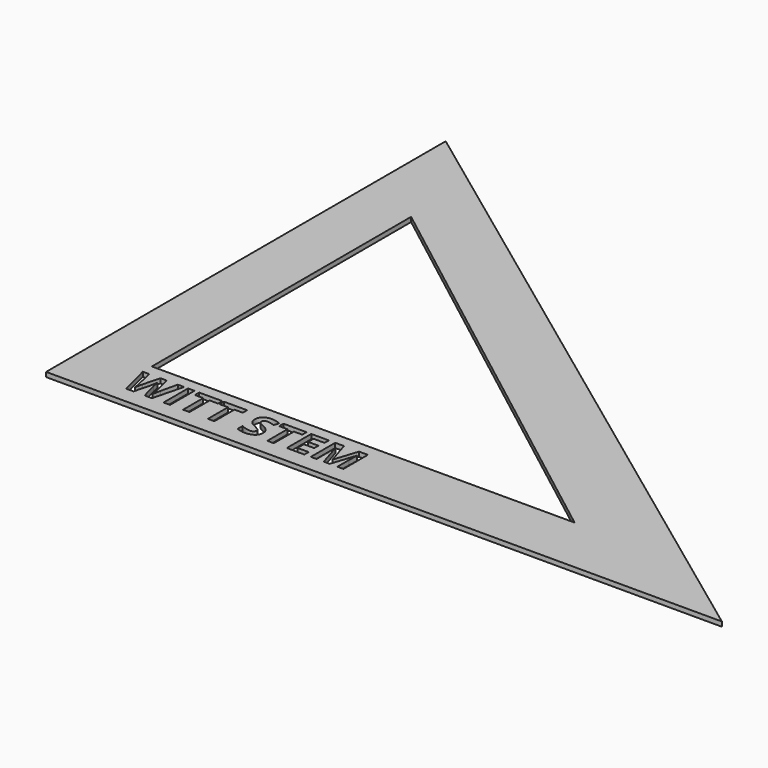
from build123d import *

# Parameters (mm, degrees)
F1_DEPTH     = 2
F2_SCALE     = 0.75
F3_TEXT_SIZE = 13.8751121122
F4_DEPTH     = 1.501


# Not quite as in the source:
# - Text() gives the source's letters only with a copy of the font that has no kerning and outlines rounded to 1/6400 em; it was checked with that copy


with BuildPart() as f1:
    # F0 (on Top) → F1 (new body)
    with BuildSketch(Plane.XY):
        Polygon((-110.3935540405, 109.5033976257), (-110.3935540405, -106.3966023743), (181.7064459595, -106.3966023743), align=None)
        Polygon((-84.9935540405, -80.9966023743), (-84.9935540405, 59.0477188125), (97.7188157638, -80.9966023743), align=None, mode=Mode.SUBTRACT)
    extrude(amount=F1_DEPTH)


with BuildPart() as f1_1:
    # F2: moved
    add(f1.part.scale(F2_SCALE))

    # F3 (on face) → F4 (cut, through all)
    with BuildSketch(Plane.XY.offset(1.5)):
        with Locations((-63.7451655304, -74.3297189474)):
            Text('WITT STEM', F3_TEXT_SIZE, font='Open Sans', font_style=FontStyle.BOLD, text_align=(TextAlign.LEFT, TextAlign.BOTTOM))
    extrude(amount=-F4_DEPTH, mode=Mode.SUBTRACT)


solid = f1_1.part
